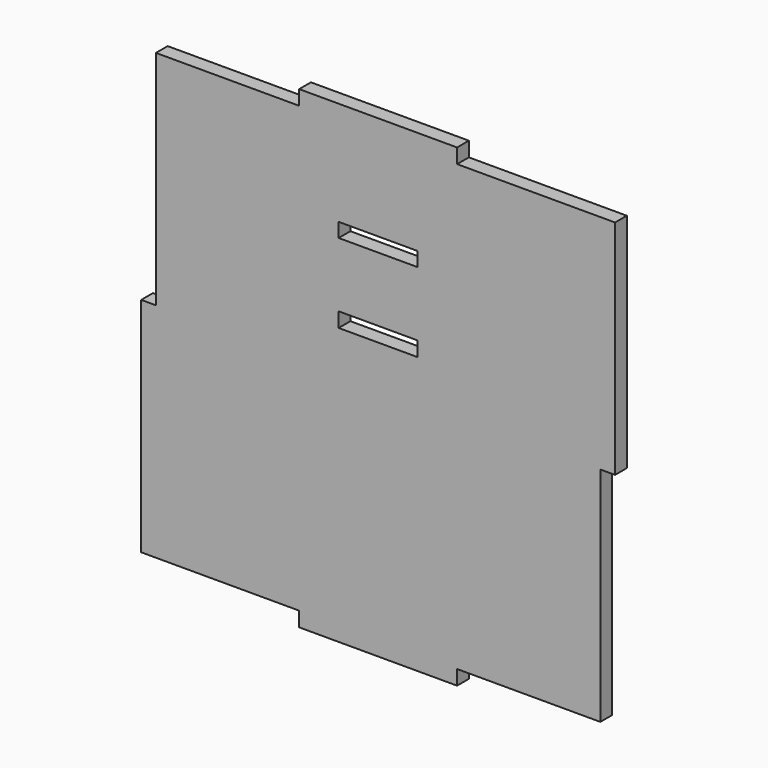
from build123d import *

# Parameters (mm, degrees)
F0_W     = 76.2
F0_H     = 76.2
F1_DEPTH = 2.3622
F2_W     = 25.4
F2_H     = 2.3622
F3_DEPTH = 2.3632
F4_W     = 2.3622
F4_H     = 35.7378
F5_DEPTH = 25.4
F6_W     = 12.7
F6_H     = 2.286
F6_H_2   = 2.3622
F7_DEPTH = 25.4


# Not quite as in the source:
# - a pattern or mirror of a feature is missing from the dataset's text; its kind, count and spacing are read off the source's solid


with BuildPart() as f1:
    # F0 (on Front) → F1 (new body)
    with BuildSketch(Plane.XZ):
        Rectangle(F0_W, F0_H)
    extrude(amount=F1_DEPTH)

    # F2 (on face) → F3 (cut, through all)
    with BuildSketch(Plane.XZ.offset(2.3622)):
        with Locations((-25.4, 36.9189)):
            Rectangle(F2_W, F2_H)
        with Locations((25.4, 36.9189)):
            Rectangle(F2_W, F2_H)
    f3 = extrude(amount=-F3_DEPTH, mode=Mode.SUBTRACT)

    # F3_copies: F3 across plane
    add(f3.mirror(Plane(origin=(0, 0, 0), x_dir=(-1, 0, 0), z_dir=(0, 0, -1))), mode=Mode.SUBTRACT)

    # F4 (on face) → F5 (cut)
    with BuildSketch(Plane.XZ.offset(2.3622)):
        with Locations((-36.9189, 17.8689)):
            Rectangle(F4_W, F4_H)
        with Locations((36.9189, -17.8689)):
            Rectangle(F4_W, F4_H)
    extrude(amount=-F5_DEPTH, mode=Mode.SUBTRACT)

    # F6 (on face) → F7 (cut)
    with BuildSketch(Plane.XZ.offset(2.3622)):
        with Locations((0, 20.2311)):
            Rectangle(F6_W, F6_H)
        with Locations((0, 7.5311)):
            Rectangle(F6_W, F6_H_2)
    extrude(amount=-F7_DEPTH, mode=Mode.SUBTRACT)


solid = f1.part
